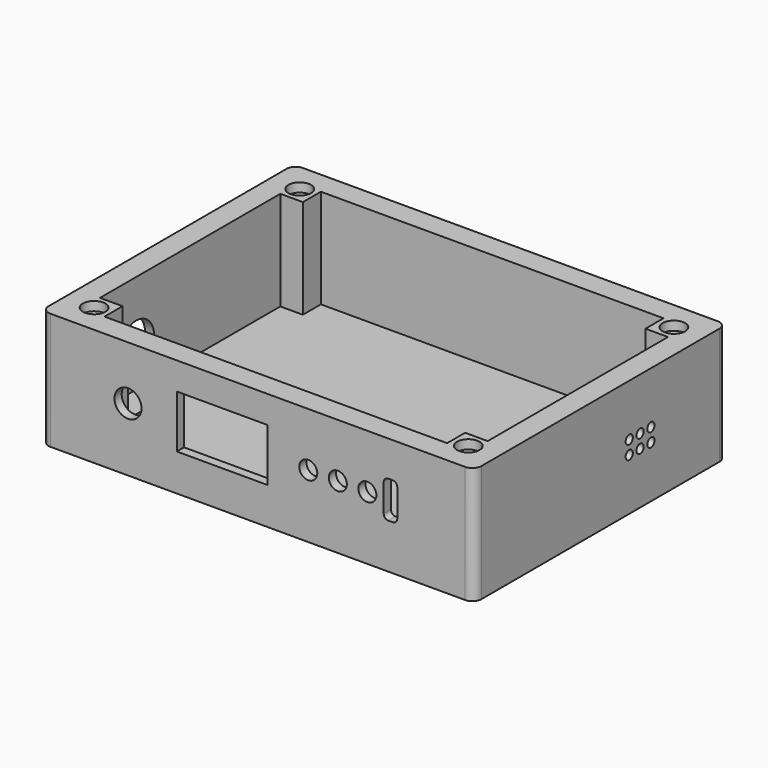
from build123d import *

# Parameters (mm, degrees)
F1_DEPTH  = 26
F3_R      = 2.5
F4_DEPTH  = 2
F5_W      = 5
F5_H      = 50
F5_W_2    = 76
F5_H_2    = 5
F6_DEPTH  = 22
F7_R      = 1
F8_DEPTH  = 5
F9_R      = 11.25
F9_R_2    = 5
F10_DEPTH = 3
F11_DEPTH = 5
F12_W     = 20.16
F12_H     = 11.72
F12_R     = 3
F12_R_2   = 2
F13_DEPTH = 5
F12_W_2   = 66
F12_H_2   = 18
F12_R_3   = 1.8
F14_DEPTH = 3
F15_DEPTH = 3
F12_R_4   = 0.8
F16_DEPTH = 1.9
F17_DEPTH = 1.9
F18_DEPTH = 1.9


# Not quite as in the source:
# - a feature names something its author has since deleted; it is built from what else it names


with BuildPart() as f1:
    # F0 (on Top) → F1 (new body)
    with BuildSketch(Plane.XY):
        with BuildLine():
            Line((46, 35), (-46, 35))
            ThreePointArc((-46, 35), (-47.4142135624, 34.4142135624), (-48, 33))
            Line((-48, 33), (-48, -33))
            ThreePointArc((-48, -33), (-47.4142135624, -34.4142135624), (-46, -35))
            Line((-46, -35), (46, -35))
            ThreePointArc((46, -35), (47.4142135624, -34.4142135624), (48, -33))
            Line((48, -33), (48, 33))
            ThreePointArc((48, 33), (47.4142135624, 34.4142135624), (46, 35))
        make_face()
    extrude(amount=F1_DEPTH)

    # F3 (on face) → F4 (cut)
    with BuildSketch(Plane.XY.offset(26)):
        with Locations((-41.5, -28.5)):
            Circle(F3_R)
        with Locations((-41.4999984205, 28.5)):
            Circle(F3_R)
        with Locations((41.5, 28.5)):
            Circle(F3_R)
        with Locations((41.5, -28.5)):
            Circle(F3_R)
    extrude(amount=-F4_DEPTH, mode=Mode.SUBTRACT)

    # F5 (on face) → F6 (cut)
    with BuildSketch(Plane.XY.offset(26)):
        with Locations((-40.5, 0)):
            Rectangle(F5_W, F5_H)
        with Locations((0, -27.5)):
            Rectangle(F5_W_2, F5_H_2)
        Rectangle(F5_W_2, F5_H)
        with Locations((0, 27.5)):
            Rectangle(F5_W_2, F5_H_2)
        with Locations((40.5, 0)):
            Rectangle(F5_W, F5_H)
    extrude(amount=-F6_DEPTH, mode=Mode.SUBTRACT)

    # F7 (on face) → F8 (cut, through all)
    with BuildSketch(Plane.YZ.offset(48)):
        with Locations((7.9999985173, 14.5000000224)):
            Circle(F7_R)
        with Locations((7.9999985173, 11.5000000224)):
            Circle(F7_R)
        with Locations((10.9999985173, 11.5000000224)):
            Circle(F7_R)
        with Locations((10.9999985173, 14.5000000224)):
            Circle(F7_R)
        with Locations((13.9999985173, 14.5000000224)):
            Circle(F7_R)
        with Locations((13.9999985173, 11.5000000224)):
            Circle(F7_R)
    extrude(amount=-F8_DEPTH, mode=Mode.SUBTRACT)

    # F9 (on face) → F10 (cut)
    with BuildSketch(Plane(origin=(-48, 0, 0), x_dir=(0, -1, 0), z_dir=(-1, 0, 0))):
        with Locations((15, 12.5000002682)):
            Circle(F9_R)
        with Locations((15, 12.5000002682)):
            Circle(F9_R_2, mode=Mode.SUBTRACT)
    extrude(amount=-F10_DEPTH, mode=Mode.SUBTRACT)

    # F9 (on face) → F11 (cut, through all)
    with BuildSketch(Plane(origin=(-48, 0, 0), x_dir=(0, -1, 0), z_dir=(-1, 0, 0))):
        with Locations((15, 12.5000002682)):
            Circle(F9_R_2)
    extrude(amount=-F11_DEPTH, mode=Mode.SUBTRACT)

    # F12 (on face) → F13 (cut, through all)
    with BuildSketch(Plane(origin=(0, -30, 0), x_dir=(-1, 0, 0), z_dir=(0, 1, 0))):
        with Locations((7.8799169147, 14.0678631142)):
            Rectangle(F12_W, F12_H)
        with Locations((28.7899169147, 14.0678631142)):
            Circle(F12_R)
        with Locations((-11.2000830853, 14.0678631142)):
            Circle(F12_R_2)
        with Locations((-17.7600830853, 14.0678631142)):
            Circle(F12_R_2)
        with Locations((-24.3100830853, 14.0678631142)):
            Circle(F12_R_2)
        with BuildLine():
            ThreePointArc((-30.9400830853, 10.9678631142), (-30.6471898665, 10.260756333), (-29.9400830853, 9.9678631142))
            Line((-29.9400830853, 9.9678631142), (-28.9400830853, 9.9678631142))
            ThreePointArc((-28.9400830853, 9.9678631142), (-28.2329763041, 10.260756333), (-27.9400830853, 10.9678631142))
            Line((-27.9400830853, 10.9678631142), (-27.9400830853, 17.1678631142))
            ThreePointArc((-27.9400830853, 17.1678631142), (-28.2329763041, 17.8749698954), (-28.9400830853, 18.1678631142))
            Line((-28.9400830853, 18.1678631142), (-29.9400830853, 18.1678631142))
            ThreePointArc((-29.9400830853, 18.1678631142), (-30.6471898665, 17.8749698954), (-30.9400830853, 17.1678631142))
            Line((-30.9400830853, 17.1678631142), (-30.9400830853, 10.9678631142))
        make_face()
    extrude(amount=-F13_DEPTH, mode=Mode.SUBTRACT)

    # F12 (on face) → F14 (cut)
    with BuildSketch(Plane(origin=(0, -30, 0), x_dir=(-1, 0, 0), z_dir=(0, 1, 0))):
        with Locations((-0.2100830853, 14.0678631142)):
            Rectangle(F12_W_2, F12_H_2)
        with BuildLine():
            Line((-28.9400830853, 9.9678631142), (-29.9400830853, 9.9678631142))
            ThreePointArc((-29.9400830853, 9.9678631142), (-30.6471898665, 10.260756333), (-30.9400830853, 10.9678631142))
            Line((-30.9400830853, 10.9678631142), (-30.9400830853, 17.1678631142))
            ThreePointArc((-30.9400830853, 17.1678631142), (-30.6471898665, 17.8749698954), (-29.9400830853, 18.1678631142))
            Line((-29.9400830853, 18.1678631142), (-28.9400830853, 18.1678631142))
            ThreePointArc((-28.9400830853, 18.1678631142), (-28.2329763041, 17.8749698954), (-27.9400830853, 17.1678631142))
            Line((-27.9400830853, 17.1678631142), (-27.9400830853, 10.9678631142))
            ThreePointArc((-27.9400830853, 10.9678631142), (-28.2329763041, 10.260756333), (-28.9400830853, 9.9678631142))
        make_face(mode=Mode.SUBTRACT)
        with Locations((-24.3100830853, 14.0678631142)):
            Circle(F12_R_2, mode=Mode.SUBTRACT)
        with Locations((-17.7600830853, 14.0678631142)):
            Circle(F12_R_2, mode=Mode.SUBTRACT)
        with Locations((-11.2000830853, 14.0678631142)):
            Circle(F12_R_2, mode=Mode.SUBTRACT)
        with Locations((30.1299169147, 7.5678631142)):
            Circle(F12_R_3, mode=Mode.SUBTRACT)
        with Locations((7.8799169147, 14.0678631142)):
            Rectangle(F12_W, F12_H, mode=Mode.SUBTRACT)
        with Locations((28.7899169147, 14.0678631142)):
            Circle(F12_R, mode=Mode.SUBTRACT)
        with Locations((-24.0500830853, 20.5678631142)):
            Circle(F12_R_3, mode=Mode.SUBTRACT)
        with Locations((30.1299169147, 20.5678631142)):
            Circle(F12_R_3, mode=Mode.SUBTRACT)
    extrude(amount=F14_DEPTH, mode=Mode.SUBTRACT)

    # F12 (on face) → F15 (cut)
    with BuildSketch(Plane(origin=(0, -30, 0), x_dir=(-1, 0, 0), z_dir=(0, 1, 0))):
        with Locations((-0.2100830853, 14.0678631142)):
            Rectangle(F12_W_2, F12_H_2)
        with BuildLine():
            Line((-28.9400830853, 9.9678631142), (-29.9400830853, 9.9678631142))
            ThreePointArc((-29.9400830853, 9.9678631142), (-30.6471898665, 10.260756333), (-30.9400830853, 10.9678631142))
            Line((-30.9400830853, 10.9678631142), (-30.9400830853, 17.1678631142))
            ThreePointArc((-30.9400830853, 17.1678631142), (-30.6471898665, 17.8749698954), (-29.9400830853, 18.1678631142))
            Line((-29.9400830853, 18.1678631142), (-28.9400830853, 18.1678631142))
            ThreePointArc((-28.9400830853, 18.1678631142), (-28.2329763041, 17.8749698954), (-27.9400830853, 17.1678631142))
            Line((-27.9400830853, 17.1678631142), (-27.9400830853, 10.9678631142))
            ThreePointArc((-27.9400830853, 10.9678631142), (-28.2329763041, 10.260756333), (-28.9400830853, 9.9678631142))
        make_face(mode=Mode.SUBTRACT)
        with Locations((-24.3100830853, 14.0678631142)):
            Circle(F12_R_2, mode=Mode.SUBTRACT)
        with Locations((-17.7600830853, 14.0678631142)):
            Circle(F12_R_2, mode=Mode.SUBTRACT)
        with Locations((-11.2000830853, 14.0678631142)):
            Circle(F12_R_2, mode=Mode.SUBTRACT)
        with Locations((30.1299169147, 7.5678631142)):
            Circle(F12_R_3, mode=Mode.SUBTRACT)
        with Locations((7.8799169147, 14.0678631142)):
            Rectangle(F12_W, F12_H, mode=Mode.SUBTRACT)
        with Locations((28.7899169147, 14.0678631142)):
            Circle(F12_R, mode=Mode.SUBTRACT)
        with Locations((-24.0500830853, 20.5678631142)):
            Circle(F12_R_3, mode=Mode.SUBTRACT)
        with Locations((30.1299169147, 20.5678631142)):
            Circle(F12_R_3, mode=Mode.SUBTRACT)
    extrude(amount=-F15_DEPTH, mode=Mode.SUBTRACT)

    # F12 (on face) → F16 (join)
    with BuildSketch(Plane(origin=(0, -30, 0), x_dir=(-1, 0, 0), z_dir=(0, 1, 0))):
        with Locations((30.1299169147, 20.5678631142)):
            Circle(F12_R_3)
        with Locations((30.1299169147, 20.5678631142)):
            Circle(F12_R_4, mode=Mode.SUBTRACT)
    extrude(amount=F16_DEPTH)

    # F12 (on face) → F17 (join)
    with BuildSketch(Plane(origin=(0, -30, 0), x_dir=(-1, 0, 0), z_dir=(0, 1, 0))):
        with Locations((30.1299169147, 7.5678631142)):
            Circle(F12_R_3)
        with Locations((30.1299169147, 7.5678631142)):
            Circle(F12_R_4, mode=Mode.SUBTRACT)
    extrude(amount=F17_DEPTH)

    # F12 (on face) → F18 (join)
    with BuildSketch(Plane(origin=(0, -30, 0), x_dir=(-1, 0, 0), z_dir=(0, 1, 0))):
        with Locations((-24.0500830853, 20.5678631142)):
            Circle(F12_R_3)
        with Locations((-24.0500830853, 20.5678631142)):
            Circle(F12_R_4, mode=Mode.SUBTRACT)
    extrude(amount=F18_DEPTH)


solid = f1.part
